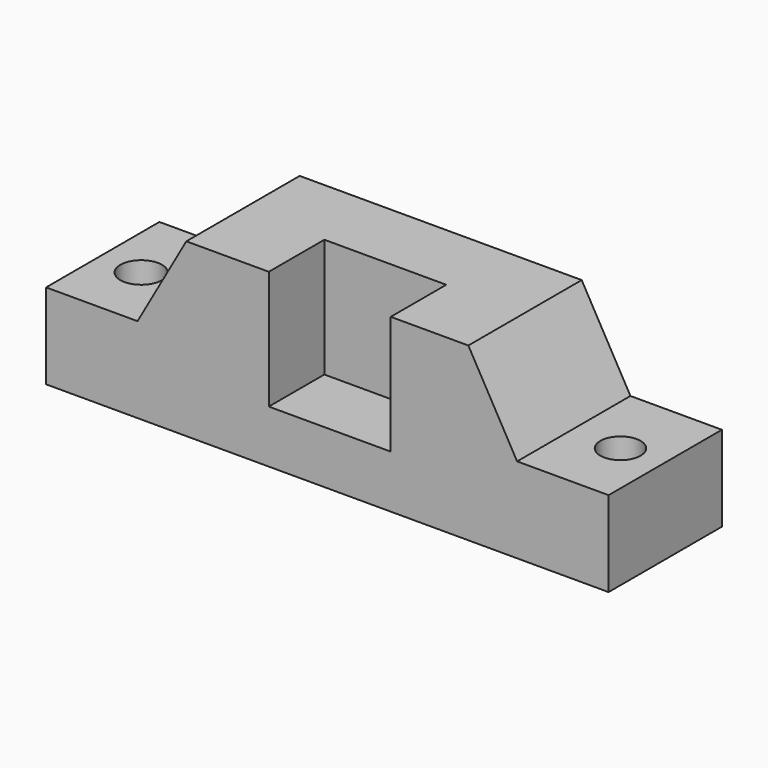
from build123d import *

# Parameters (mm, degrees)
F1_DEPTH = 25.4
F2_W     = 21.8606553972
F2_H     = 22.4436074495
F3_DEPTH = 12.446
F4_R     = 3.7327062706
F4_R_2   = 3.6053518758
F5_DEPTH = 25.4


# Not quite as in the source:
# - ends of sketch curves that miss each other by under 0.0002 mm in the source are joined


with BuildPart() as f1:
    # F0 (on Front) → F1 (new body)
    with BuildSketch(Plane.XZ):
        Polygon((25.2813665716, 30.7506565005), (-8.463e-07, 30.7506565005), (-8.463e-07, 0), (50.4252426326, 0), (50.4252426326, 15.3024597093), (34.0256324557, 15.3024597093), align=None)
        Polygon((-8.463e-07, 0), (-8.463e-07, 30.7506565005), (-25.2813665716, 30.7506565005), (-34.0256324557, 15.3024597093), (-50.4252426326, 15.3024597093), (-50.4252426326, 0), align=None)
    extrude(amount=F1_DEPTH)

    # F2 (on face) → F3 (cut)
    with BuildSketch(Plane.XZ.offset(25.4)):
        with Locations((0.4372131079, 20.6947550178)):
            Rectangle(F2_W, F2_H)
    extrude(amount=-F3_DEPTH, mode=Mode.SUBTRACT)

    # F4 (on face) → F5 (cut)
    with BuildSketch(Plane.XY.offset(15.3024597093)):
        with Locations((-42.8468845785, -13.5536063462)):
            Circle(F4_R)
        with Locations((42.8468845785, -13.2621303201)):
            Circle(F4_R_2)
    extrude(amount=-F5_DEPTH, mode=Mode.SUBTRACT)


solid = f1.part
